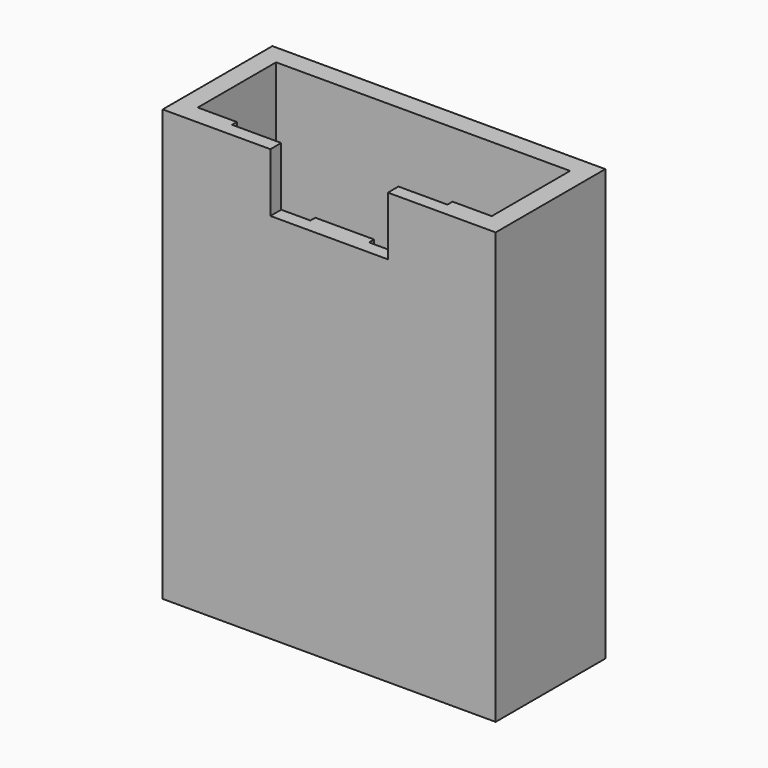
from build123d import *

# Parameters (mm, degrees)
F1_DEPTH = 11.1125
F2_W     = 6.35
F2_H     = 0.5200478494
F2_H_2   = 0.4923428655
F3_DEPTH = 32.54375
F5_DEPTH = 2.38225
F6_W     = 9.525
F6_H     = 4.7625
F7_DEPTH = 3.175


# Not quite as in the source:
# - a feature names something its author has since deleted; it is built from what else it names


with BuildPart() as f1:
    # F0 (on Front) → F1 (new body)
    with BuildSketch(Plane.XZ):
        Polygon((-30.725677704, 46.6747839019), (-42.3673422778, 46.6747839019), (-42.3673422778, 11.7497839019), (-15.3798422778, 11.7497839019), (-15.3798422778, 46.6747839019), align=None)
    extrude(amount=F1_DEPTH)

    # F2 (on face) → F3 (cut)
    with BuildSketch(Plane.XY.offset(46.6747839019)):
        Polygon((-16.9673422778, -9.525), (-16.9673422778, -1.5875), (-20.1423422778, -1.5875), (-40.7925422778, -1.5875), (-40.7925422778, -9.525), (-37.6187860966, -9.525), (-31.2687860966, -9.525), (-26.4923422778, -9.525), (-20.1423422778, -9.525), align=None)
        with Locations((-23.3173422778, -9.7850239247)):
            Rectangle(F2_W, F2_H)
        with Locations((-34.4437860966, -9.7711714327)):
            Rectangle(F2_W, F2_H_2)
    extrude(amount=-F3_DEPTH, mode=Mode.SUBTRACT)

    # F4 (on face) → F5 (cut, through all)
    with BuildSketch(Plane.XY.offset(14.1310339019)):
        with BuildLine():
            ThreePointArc((-34.4437860966, -9.525), (-32.1987220663, -8.5950640303), (-31.2687860966, -6.35))
            ThreePointArc((-31.2687860966, -6.35), (-36.6888501268, -4.1049359697), (-34.4437860966, -9.525))
        make_face()
    extrude(amount=-F5_DEPTH, mode=Mode.SUBTRACT)

    # F6 (on face) → F7 (cut)
    with BuildSketch(Plane.XZ.offset(11.1125)):
        with Locations((-28.8735922778, 44.2935339019)):
            Rectangle(F6_W, F6_H)
    extrude(amount=-F7_DEPTH, mode=Mode.SUBTRACT)


solid = f1.part
